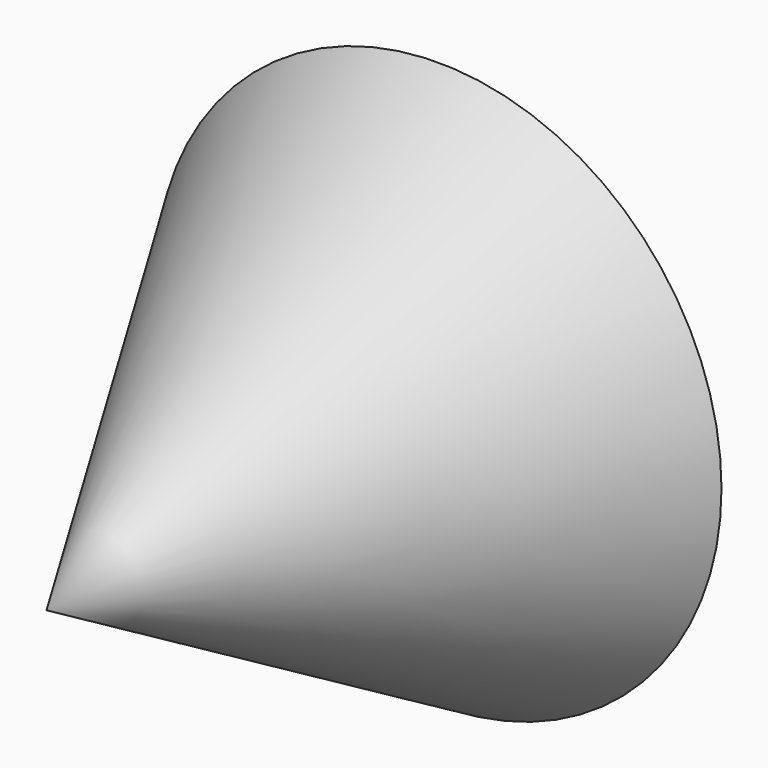
from build123d import *

# Parameters (mm, degrees)
F0_R = 57.4715007944


# Not quite as in the source:
# - an extrude whose draft closes it to a point is written as a loft to that point


with BuildPart() as f1:
    # F0 (on Front) → F1 section 0
    with BuildSketch(Plane.XZ, mode=Mode.PRIVATE) as f1_s0:
        with Locations((0, -2.1279256325)):
            Circle(F0_R)
    loft([f1_s0.sketch, Vertex(0, -99.5435593631, -2.1279256325)], ruled=True)


solid = f1.part
